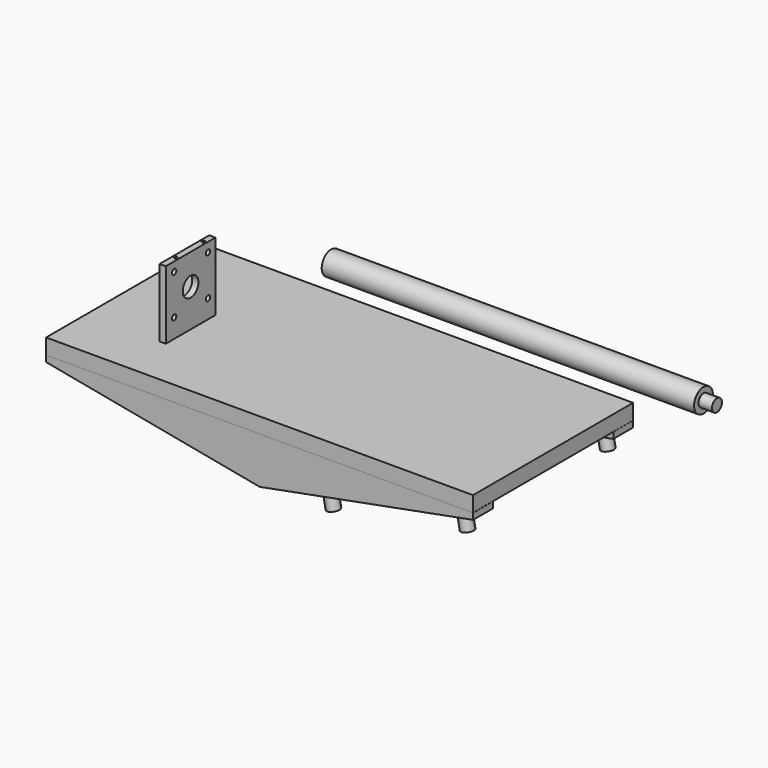
from build123d import *

# Parameters (mm, degrees)
F1_DEPTH  = 40
F2_R      = 5
F3_DEPTH  = 10
F4_R      = 10
F5_DEPTH  = 25
F6_R      = 10
F7_DEPTH  = 25
F8_W      = 687.9218816757
F8_H      = 322.3598301411
F9_DEPTH  = 25
F11_DEPTH = 40
F12_R     = 10
F13_DEPTH = 25
F14_W     = 10
F14_H     = 100
F14_R     = 2.5
F15_DEPTH = 110
F16_R     = 4.3389942533
F16_R_2   = 15.7440759203
F17_DEPTH = 66
F20_R     = 18.9932010267
F21_DEPTH = 600
F22_R     = 10
F23_DEPTH = 21.7


# Not quite as in the source:
# - the program builds the solid bodies; features that only make, move or delete a surface that nothing else refers to are left out


with BuildPart() as f1:
    # F0 (on Front) → F1 (new body)
    with BuildSketch(Plane.XZ):
        Polygon((343.9113257804, 0), (-343.9113257804, 0), (-343.9113257804, -10), (0, -75), (343.9113257804, -10), align=None)
    extrude(amount=F1_DEPTH)

    # F2 (on face) → F3 (cut)
    with BuildSketch(Plane.XY):
        with Locations((-264.9109515785, -20)):
            Circle(F2_R)
        with Locations((-104.1895777367, -20)):
            Circle(F2_R)
        with Locations((104.1895777367, -20)):
            Circle(F2_R)
        with Locations((264.9109515785, -20)):
            Circle(F2_R)
    extrude(amount=-F3_DEPTH, mode=Mode.SUBTRACT)

    # F4 (on face) → F5 (join)
    with BuildSketch(Plane(origin=(-13.6862670464, 0, -72.4132653061), x_dir=(0.9826037879, 0, -0.1857142857), z_dir=(-0.1857142857, 0, -0.9826037879))):
        with Locations((-306.0714285714, 20)):
            Circle(F4_R)
        with Locations((-86.0714285714, 20)):
            Circle(F4_R)
    extrude(amount=F5_DEPTH)

    # F6 (on face) → F7 (join)
    with BuildSketch(Plane(origin=(13.6862670464, 0, -72.4132653061), x_dir=(0.9826037879, 0, 0.1857142857), z_dir=(0.1857142857, 0, -0.9826037879))):
        with Locations((306.0714285714, 20)):
            Circle(F6_R)
        with Locations((86.0714285714, 20)):
            Circle(F6_R)
    extrude(amount=F7_DEPTH)


with BuildPart() as f9:
    # F8 (on Top) → F9 (new body)
    with BuildSketch(Plane.XY):
        with Locations((-0.2017915249, -161.1799150705)):
            Rectangle(F8_W, F8_H)
    extrude(amount=F9_DEPTH)


with BuildPart() as f11:
    # F10 (on face) → F11 (new body)
    with BuildSketch(Plane.XZ.offset(322.3598301411)):
        Polygon((344.0105558954, 0), (-343.9113257804, 0), (-343.9113257804, -10), (0, -75), (344.0105558954, -10), align=None)
    extrude(amount=-F11_DEPTH)

    # F12 (on face) → F13 (join)
    with BuildSketch(Plane(origin=(13.6825914381, 0, -72.4147059495), x_dir=(0.9826135622, 0, 0.1856625631), z_dir=(0.1856625631, 0, -0.9826135622))):
        with Locations((306.0753077668, 302.3598301411)):
            Circle(F12_R)
        with Locations((86.0753077668, 302.3598301411)):
            Circle(F12_R)
    extrude(amount=F13_DEPTH)


with BuildPart() as f15:
    # F14 (on face) → F15 (new body)
    with BuildSketch(Plane.XY.offset(25)):
        with Locations((-220.8246585727, -191.7345849391)):
            Rectangle(F14_W, F14_H)
        with Locations((-220.8246585727, -215.2414023876)):
            Circle(F14_R, mode=Mode.SUBTRACT)
        with Locations((-220.8246585727, -159.5595628023)):
            Circle(F14_R, mode=Mode.SUBTRACT)
    extrude(amount=F15_DEPTH)

    # F16 (on face) → F17 (cut)
    with BuildSketch(Plane.YZ.offset(-215.8246585727)):
        with Locations((-156.7345849391, 120)):
            Circle(F16_R)
        with Locations((-156.7345849391, 55)):
            Circle(F16_R)
        with Locations((-224.8520583823, 120)):
            Circle(F16_R)
        with Locations((-224.8520583823, 55.5403646578)):
            Circle(F16_R)
        with Locations((-191.7345849391, 85.5679959059)):
            Circle(F16_R_2)
    extrude(amount=-F17_DEPTH, mode=Mode.SUBTRACT)


with BuildPart() as f21:
    # F20 (on offset) → F21 (new body)
    with BuildSketch(Plane.YZ.offset(-108.8246585727)):
        with Locations((-42.3773415387, 93.7410518527)):
            Circle(F20_R)
    extrude(amount=F21_DEPTH)

    # F22 (on face) → F23 (join)
    with BuildSketch(Plane.YZ.offset(491.1753414273)):
        with Locations((-42.3773415387, 93.7410518527)):
            Circle(F22_R)
    extrude(amount=F23_DEPTH)


solid = Compound([f1.part, f9.part, f11.part, f15.part, f21.part])
